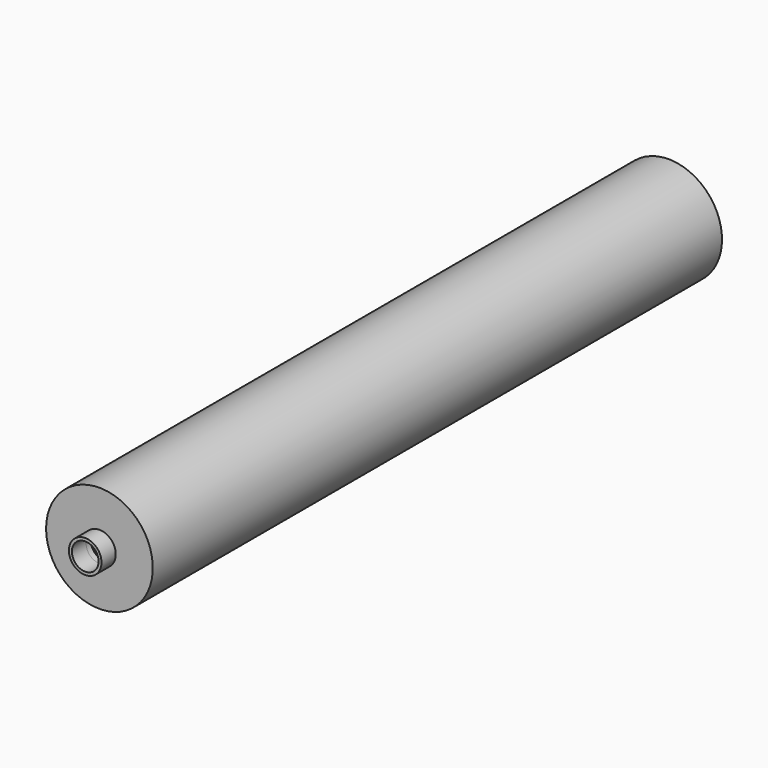
from build123d import *

# Parameters (mm, degrees)
F0_R     = 2.75
F0_R_2   = 2.25
F1_DEPTH = 3
F2_R     = 9
F3_DEPTH = 120
F4_T     = 1
F5_DEPTH = 25


# Not quite as in the source:
# - a shell that OpenCascade refuses in one call is made with other operations: the cavity is built on its own and cut out


with BuildPart() as f1:
    # F0 (on Front) → F1 (new body)
    with BuildSketch(Plane.XZ):
        Circle(F0_R)
        Circle(F0_R_2, mode=Mode.SUBTRACT)
    extrude(amount=F1_DEPTH)

    # F2 (on face) → F3 (join)
    with BuildSketch(Plane(origin=(0, 0, 0), x_dir=(-1, 0, 0), z_dir=(0, 1, 0))):
        Circle(F2_R)
    extrude(amount=F3_DEPTH)

    # F4: shell of thickness 1, made by hand


with BuildPart() as f4_core1:
    # F4_t2: copy of F1
    add(f1.part)

    # the walls: a layer under each face that stays
    f4_faces = [f4_core1.faces().sort_by_distance(p)[0] for p in [
        (9, 60, 0),
        (6, 0, -6),
        (-2.75, -1.5, 0),
        (-1.8333333333, -3, -1.8333333333),
        (-2.25, -1.5, 0),
        (0, 0, 0),
    ]]
    thicken(f4_faces, amount=-F4_T, mode=Mode.SUBTRACT)

    # F4_s3 → F4_t4 (revolve, cut)
    with BuildSketch(Plane.XY):
        Polygon((2.76, -0.01), (2.75, 1), (1.75, 1), (1.75, 0), align=None)
    revolve(axis=Axis((0, 0, 0), (0, -1, 0)), mode=Mode.SUBTRACT)

    # F4_s5 → F4_t6 (revolve, cut)
    with BuildSketch(Plane.XY):
        Polygon((2.24, -0.01), (3.25, 0), (3.25, 1), (2.25, 1), align=None)
    revolve(axis=Axis((0, 0, 0), (0, -1, 0)), mode=Mode.SUBTRACT)


with BuildPart() as f1_1:
    add(f1.part)

    # what is left inside the walls is the cavity
    f4_cavity = [f4_core1.part.solids().sort_by_distance(p)[0] for p in [
        (7.99, 80.333333, 0),
    ]]
    add(f4_cavity, mode=Mode.SUBTRACT)

    # F0 (on Front) → F5 (cut)
    with BuildSketch(Plane.XZ):
        Circle(F0_R_2)
    extrude(amount=-F5_DEPTH, mode=Mode.SUBTRACT)


solid = f1_1.part
